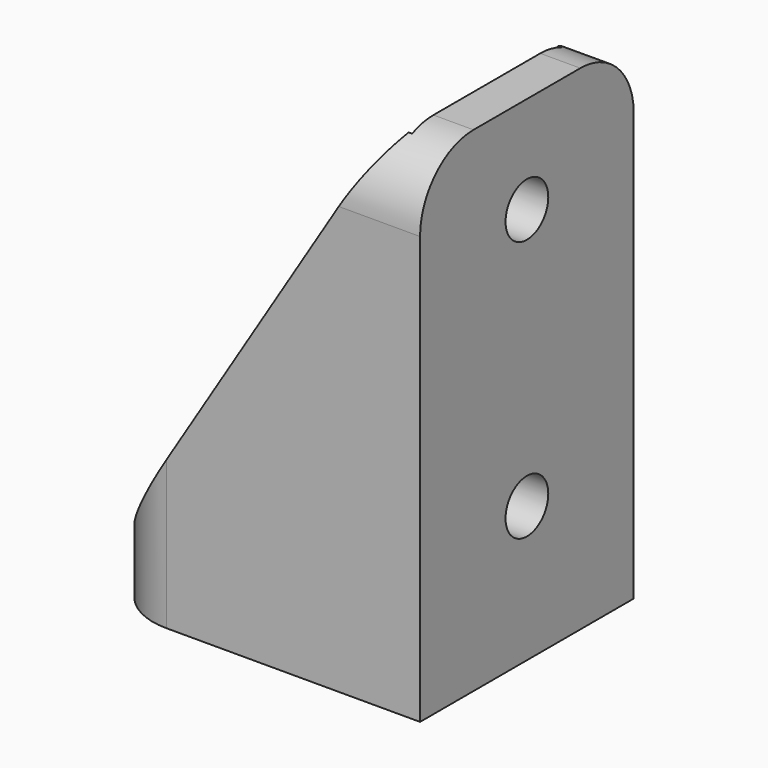
from build123d import *

# Parameters (mm, degrees)
F1_DEPTH        = 3
F2_W            = 3
F2_H            = 20
F3_DEPTH        = 34
F5_DEPTH        = 3
F8_D            = 4
F10_D           = 3.3
F10_CSINK_D     = 7
F10_CSINK_ANGLE = 90
F11_T1_DEPTH    = 28
F11_T3_DEPTH    = 28


# Not quite as in the source:
# - a fillet or chamfer that OpenCascade refuses, or shapes differently, is made with other operations: its cross-section is extruded or revolved along the edge and cut away or added


with BuildPart() as f1:
    # F0 (on Top) → F1 (new body)
    with BuildSketch(Plane.XY):
        Polygon((0, 10), (0, 0), (0, -10), (24, -10), (24, 0), (24, 10), align=None)
    extrude(amount=F1_DEPTH)

    # F2 (on face) → F3 (join)
    with BuildSketch(Plane.XY.offset(3)):
        with Locations((22.5, 0)):
            Rectangle(F2_W, F2_H)
    extrude(amount=F3_DEPTH)

    # F4 (on face) → F5 (join)
    with BuildSketch(Plane.XZ.offset(10)):
        Polygon((21, 3), (21, 37), (0, 3), align=None)
    extrude(amount=-F5_DEPTH)

    # F6: F1 across plane


with BuildPart() as f1_1:
    add(f1.part)
    add(f1.part.mirror(Plane.XZ))

    # F8 (through all)
    with Locations(Plane(origin=(21, 0, 0), x_dir=(0, -1, 0), z_dir=(-1, 0, 0))):
        with Locations((0, 10.16), (0, 29.718)):
            Hole(F8_D / 2)

    # F10 (through all)
    with Locations(Plane.XY.offset(3)):
        with Locations((10.5, 0)):
            CounterSinkHole(F10_D / 2, F10_CSINK_D / 2, counter_sink_angle=F10_CSINK_ANGLE)

    # F11: fillet of radius 5 on 4 edges, made by hand

    # F11_s2 → F11_t1 (cut)
    with BuildSketch(Plane.XY.offset(-12.5)):
        with BuildLine():
            ThreePointArc((0, -5), (1.4644660941, -8.5355339059), (5, -10))
            Line((5, -10), (0, -10))
            Line((0, -10), (0, -5))
        make_face()
        with BuildLine():
            ThreePointArc((0, 5), (1.4644660941, 8.5355339059), (5, 10))
            Line((5, 10), (0, 10))
            Line((0, 10), (0, 5))
        make_face()
    extrude(amount=F11_T1_DEPTH, mode=Mode.SUBTRACT)

    # F11_s4 → F11_t3 (cut)
    with BuildSketch(Plane.YZ.offset(8.5)):
        with BuildLine():
            ThreePointArc((-10, 32), (-8.5355339059, 35.5355339059), (-5, 37))
            Line((-5, 37), (-10, 37))
            Line((-10, 37), (-10, 32))
        make_face()
        with BuildLine():
            ThreePointArc((10, 32), (8.5355339059, 35.5355339059), (5, 37))
            Line((5, 37), (10, 37))
            Line((10, 37), (10, 32))
        make_face()
    extrude(amount=F11_T3_DEPTH, mode=Mode.SUBTRACT)


solid = f1_1.part
